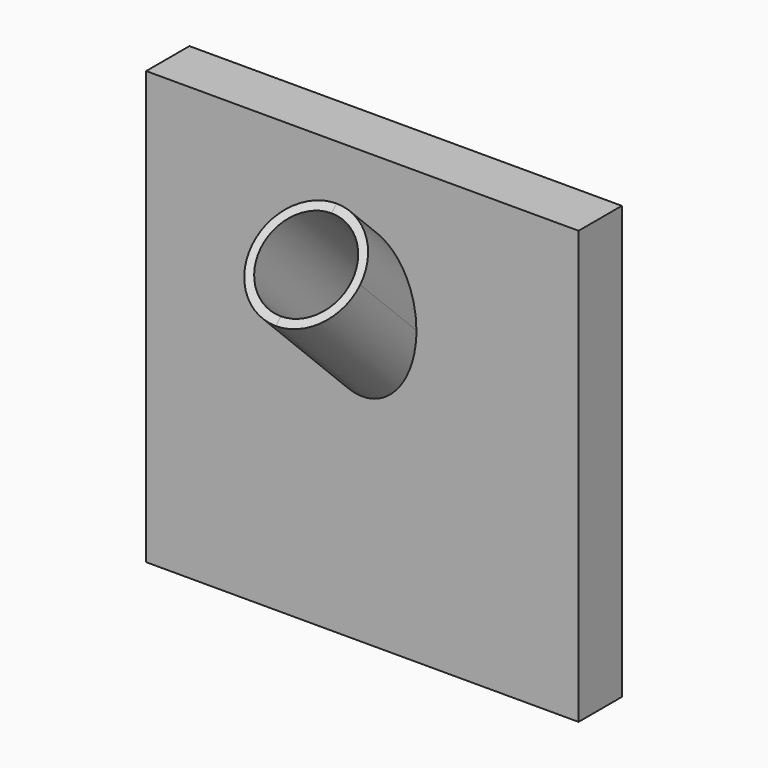
from build123d import *

# Parameters (mm, degrees)
F0_W     = 200
F0_H     = 200
F1_DEPTH = 25
F3_DEPTH = 25
F4_R     = 25
F5_REACH = 228.5588830885
F7_REACH = 193.2035440291
F8_R     = 21
F9_DEPTH = 101.0840931723


with BuildPart() as f1:
    # F0 (on Front) → F1 (new body)
    with BuildSketch(Plane.XZ):
        Rectangle(F0_W, F0_H)
    extrude(amount=F1_DEPTH)

    # F2 (on Right) → F3 (join)
    with BuildSketch(Plane.YZ):
        Polygon((-74.9957839266, 48.9940974972), (-25, 0), (-25, 70.0059030005), (-40, 84.7053717305), align=None)
    extrude(amount=F3_DEPTH)

    f5_end = Plane(origin=(-0.5719458586, -25, -1.601583452), x_dir=(0, 0, -1), z_dir=(0, -1, 0))
    # F4 (on face) → F5 (join, up to a plane its end follows)
    with BuildSketch(Plane(origin=(0, -62.7487350002, 61.4915378653), x_dir=(1, 0, 0), z_dir=(0, -0.7142254847, 0.6999156785))):
        with Locations((0, 7.5021080367)):
            Circle(F4_R)
    f5_long = extrude(amount=-F5_REACH, mode=Mode.PRIVATE)
    add(split(f5_long, bisect_by=f5_end, keep=Keep.TOP, mode=Mode.PRIVATE))

    f7_end = Plane(origin=(-0.1977552343, -25, -2.9660534924), x_dir=(0, 0, -1), z_dir=(0, -1, 0))
    # F6 (on face) → F7 (cut, up to a plane its end follows)
    with BuildSketch(Plane(origin=(0, -62.7487350002, 61.4915378653), x_dir=(1, 0, 0), z_dir=(0, -0.7142254847, 0.6999156785))):
        with BuildLine():
            ThreePointArc((0, 32.5021080367), (17.6776695297, 25.1797775664), (25, 7.5021080367))
            Line((25, 7.5021080367), (25, 32.5021080367))
            Line((25, 32.5021080367), (0, 32.5021080367))
        make_face()
        with BuildLine():
            ThreePointArc((25, 7.5021080367), (17.6776695297, -10.175561493), (0, -17.4978919633))
            Line((0, -17.4978919633), (25, -17.4978919633))
            Line((25, -17.4978919633), (25, 7.5021080367))
        make_face()
    f7_long = extrude(amount=-F7_REACH, mode=Mode.PRIVATE)
    add(split(f7_long, bisect_by=f7_end, keep=Keep.TOP, mode=Mode.PRIVATE), mode=Mode.SUBTRACT)

    # F8 (on face) → F9 (cut, through all)
    with BuildSketch(Plane(origin=(0, -62.7487350002, 61.4915378653), x_dir=(1, 0, 0), z_dir=(0, -0.7142254847, 0.6999156785))):
        with Locations((0, 7.5021080367)):
            Circle(F8_R)
    extrude(amount=-F9_DEPTH, mode=Mode.SUBTRACT)


solid = f1.part
